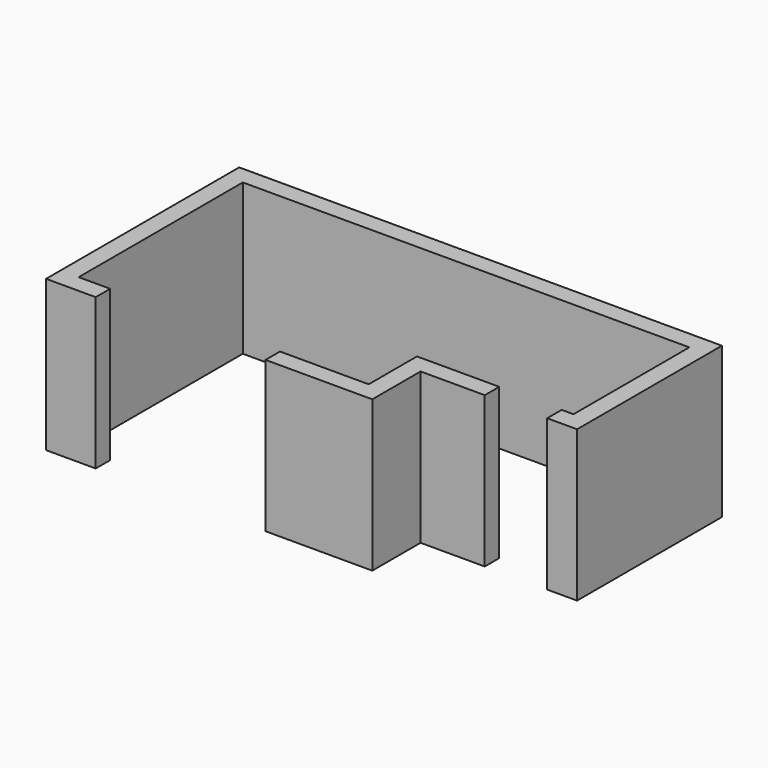
from build123d import *

# Parameters (mm, degrees)
F1_DEPTH = 2500


# Not quite as in the source:
# - a feature of the source that left no trace in its solid (it failed there, or was rolled back) is left out


with BuildPart() as f1:
    # F0 (on Top) → F1 (new body)
    with BuildSketch(Plane.XY):
        Polygon((3971.811182797, 1693.5292053778), (-4028.188817203, 1693.5292053778), (-4028.188817203, -2306.4707946222), (-3206.0170832425, -2306.4707946222), (-3206.0170832425, -2006.4707946222), (-3728.188817203, -2006.4707946222), (-3728.188817203, 1393.5292053778), (3671.811182797, 1393.5292053778), (3671.811182797, -1006.4707946222), (3475.8865002422, -1006.4707946222), (3475.8865002422, -1306.4707946222), (3971.811182797, -1306.4707946222), align=None)
    extrude(amount=F1_DEPTH)


with BuildPart() as f1b:
    # F0 (on Top) → F1, piece 2 (new body)
    with BuildSketch(Plane.XY):
        Polygon((1377.9044771042, -1306.4707946222), (2441.3231871367, -1306.4707946222), (2441.3231871367, -1006.4707946222), (1077.9044771042, -1006.4707946222), (1077.9044771042, -2006.4707946222), (-391.8183739582, -2006.4707946222), (-391.8183739582, -2306.4707946222), (1377.9044771042, -2306.4707946222), align=None)
    extrude(amount=F1_DEPTH)


solid = Compound([f1.part, f1b.part])
